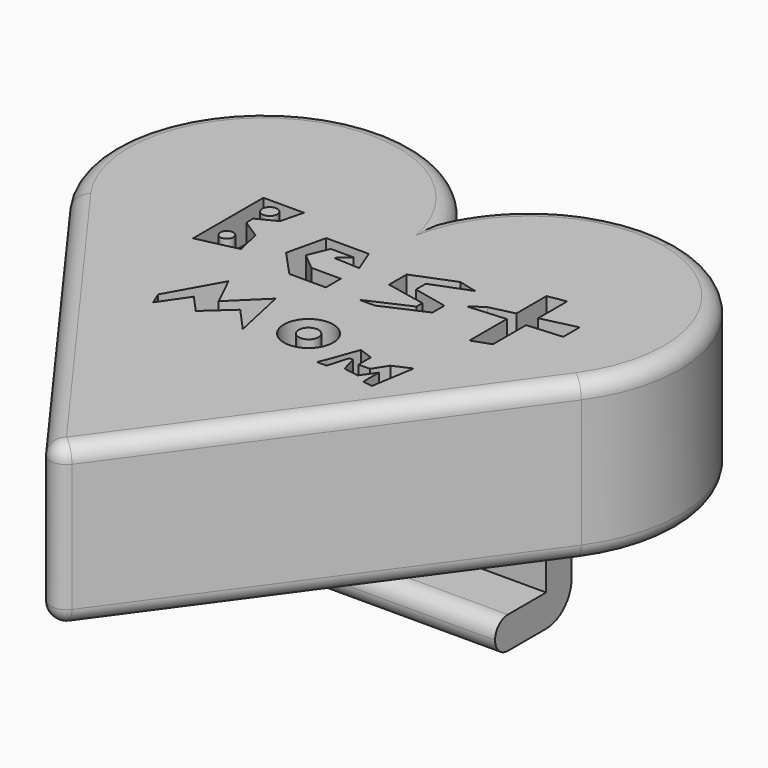
from build123d import *

# Parameters (mm, degrees)
F1_DEPTH  = 12.7
F2_R      = 1.27
F3_W      = 33.0184467606
F3_H      = 7.62
F4_DEPTH  = 6.35
F6_DEPTH  = 5.08
F7_R      = 2.54
F8_R      = 1.26999
F10_R     = 0.5243142603
F10_R_2   = 0.598941464
F10_R_3   = 1.9572905624
F10_R_4   = 0.79146579
F11_DEPTH = 2.54


# Not quite as in the source:
# - a fillet or chamfer is up to 0.001 mm smaller than in the source, because OpenCascade refuses the exact size
# - a feature of the source that left no trace in its solid (it failed there, or was rolled back) is left out


with BuildPart() as f1:
    # F0 (on Top) → F1 (new body)
    with BuildSketch(Plane.XY):
        Polygon((0, -27.94), (0, 0), (-20.32, 0), align=None)
        with BuildLine():
            Line((-20.32, 0), (0, 0))
            Line((0, 0), (-13.111957335, 18.7258157324))
            ThreePointArc((-13.111957335, 18.7258157324), (-21.7665907667, 11.3070168981), (-20.32, 0))
        make_face()
        with BuildLine():
            Line((0, 0), (0, 12.7))
            ThreePointArc((0, 12.7), (-5.5495799526, 17.902795111), (-13.111957335, 18.7258157324))
            Line((-13.111957335, 18.7258157324), (0, 0))
        make_face()
        with BuildLine():
            ThreePointArc((13.111957335, 18.7258157324), (5.5495799526, 17.902795111), (0, 12.7))
            Line((0, 12.7), (0, 0))
            Line((0, 0), (13.111957335, 18.7258157324))
        make_face()
        with BuildLine():
            Line((13.111957335, 18.7258157324), (0, 0))
            Line((0, 0), (20.32, 0))
            ThreePointArc((20.32, 0), (21.7665907667, 11.3070168981), (13.111957335, 18.7258157324))
        make_face()
        Polygon((20.32, 0), (0, 0), (0, -27.94), align=None)
    extrude(amount=F1_DEPTH)

    # F2
    f2_edges = [f1.edges().sort_by_distance(p)[0] for p in [
        (0, -27.94, 6.35),
    ]]
    fillet(f2_edges, radius=F2_R)

    # F3 (on face) → F4 (join)
    with BuildSketch(Plane(origin=(0, 0, 0), x_dir=(1, 0, 0), z_dir=(0, 0, -1))):
        Rectangle(F3_W, F3_H)
    extrude(amount=F4_DEPTH)

    # F5 (on face) → F6 (cut)
    with BuildSketch(Plane.XZ.offset(3.81)):
        Polygon((-16.5092233803, -3.81), (0, -3.81), (16.5092233803, -3.81), (16.5092233803, 0), (-16.5092233803, 0), align=None)
    extrude(amount=-F6_DEPTH, mode=Mode.SUBTRACT)

    # F7
    f7_edges = [f1.edges().sort_by_distance(p)[0] for p in [
        (0, 3.81, -6.35),
    ]]
    fillet(f7_edges, radius=F7_R)

    # F8 (radius 1.27 in the source; OpenCascade refuses exactly that, so slightly less here)
    f8_edges = [f1.edges().sort_by_distance(p)[0] for p in [
        (0, -3.81, -3.81),
        (0, -3.81, -6.35),
        (-10.673547, -13.263872, 12.7),
        (10.673547, -13.263872, 0),
    ]]
    fillet(f8_edges, radius=F8_R)

    # F10 (on face) → F11 (cut)
    with BuildSketch(Plane.XY.offset(12.7)):
        Polygon((-7.3335906491, 6.9943653395), (-10.5627283372, 6.9943653395), (-10.5627283372, 0), (-7.3335906491, 0.7349486114), (-7.79060311, 2.7429205143), (-9.3015888706, 3.7297289819), (-9.3015888706, 4.4142501429), (-7.79060311, 5.1843370311), align=None)
        with Locations((-9.2159248888, 1.6810059315)):
            Circle(F10_R, mode=Mode.SUBTRACT)
        with Locations((-9.0948464349, 5.7926201262)):
            Circle(F10_R_2, mode=Mode.SUBTRACT)
        Polygon((-5.2438098937, -3.1229529995), (-7.5429510325, -7.2372052819), (-7.1194251068, -8.2657681778), (-5.6228582704, -6.0908141027), (-4.3273653508, -7.5203236143), (-2.2791281808, -5.6641087867), (-0.5245208158, -7.6002273709), (-1.4925802825, -3.1229529995), (-4.0337359533, -5.60360495), align=None)
        Polygon((-2.0902381511, 3.4230099991), (0, 3.3229410183), (-0.7406336372, 5.1936786622), (-4.1223512962, 5.1936786622), (-4.841865506, 2.0997666288), (-2.8991762083, 0), (0, 0), (0, 1.4977937099), (-2.3469333537, 1.4977937099), (-3.6731935106, 2.6101409458), (-2.9886723496, 4.2358790524), (-1.1918039527, 4.2358790524), align=None)
        Polygon((7.5416904874, 5.4201777093), (6.0734692961, 5.7895942591), (2.8356553521, 4.4944682159), (2.8356553521, 2.7429205143), (6.001518108, 2.0997666288), (6.001518108, 1.4977937099), (2.6644766331, 0), (3.9051719941, 0), (7.2849951684, 1.4977937099), (7.2849951684, 2.6820923667), (4.5469105244, 3.281048499), (4.5469105244, 4.2650480755), align=None)
        Polygon((12.8831379116, 3.8117669891), (11.4310486242, 3.702860409), (11.4310486242, 0), (12.8831379116, 0.5112900399), align=None)
        Polygon((11.4310486242, 3.702860409), (11.4310486242, 4.6575730793), (9.4949305058, 4.2020159308), (8.4058633074, 3.4759717528), align=None)
        Polygon((12.8831379116, 7.8927418217), (11.4310486242, 7.6507278718), (11.4310486242, 4.6575730793), (12.8831379116, 4.999241105), align=None)
        Polygon((15.6663097441, 5.6541049853), (12.8831379116, 4.999241105), (12.8831379116, 3.8117669891), (15.6663097441, 4.0205046535), align=None)
        Polygon((12.8831379116, 4.999241105), (11.4310486242, 4.6575730793), (11.4310486242, 3.702860409), (12.8831379116, 3.8117669891), align=None)
        Polygon((6.9560511038, -5.2067907527), (6.0911364853, -7.59802619), (5.8446256444, -8.1831160933), (6.6077862866, -8.1831160933), (7.0911212824, -6.5296017565), (7.3963850737, -6.5296017565), (7.727087941, -7.801536005), (8.9402683079, -8.0050453544), (9.7322071764, -6.8857432343), (9.7322071764, -8.4376684573), (10.517465882, -8.5646957159), (11.0771171749, -5.1050363109), (9.7034284845, -5.7155638933), (8.9911455289, -6.8348660134), (8.0683877672, -6.8348660134), (8.0683877672, -5.6091251385), align=None)
        with Locations((3.0384953134, -5.5120550096)):
            Circle(F10_R_3)
        with Locations((3.0384953134, -5.5120550096)):
            Circle(F10_R_4, mode=Mode.SUBTRACT)
    extrude(amount=-F11_DEPTH, mode=Mode.SUBTRACT)


solid = f1.part
